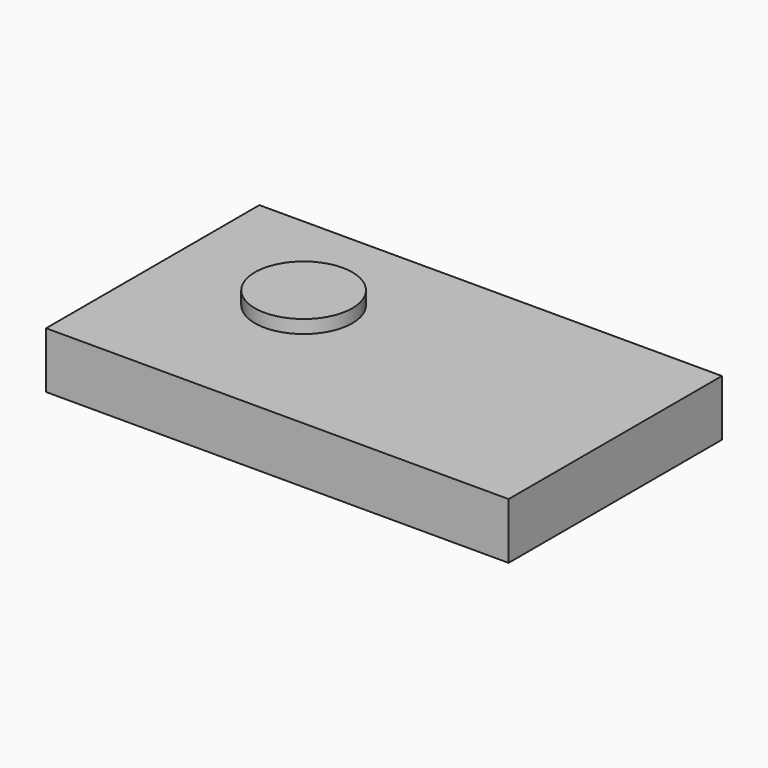
from build123d import *

# Parameters (mm, degrees)
F0_W     = 70
F0_H     = 40.35
F1_DEPTH = 8.5
F2_T     = -2
F3_R     = 7.375
F4_DEPTH = 2
F3_R_2   = 2.3617937204
F3_R_3   = 2.35
F5_DEPTH = 6


with BuildPart() as f1:
    # F0 (on Top) → F1 (new body)
    with BuildSketch(Plane.XY):
        with Locations((0, 20.175)):
            Rectangle(F0_W, F0_H)
    extrude(amount=F1_DEPTH)

    # F2
    f2_openings = [f1.faces().sort_by_distance(p)[0] for p in [
        (0, 20.175, 0),
    ]]
    offset(amount=F2_T, openings=f2_openings)


with BuildPart() as f4:
    # F3 (on face) → F4 (new body)
    with BuildSketch(Plane(origin=(0, 0, 6.5), x_dir=(1, 0, 0), z_dir=(0, 0, -1))):
        with Locations((-14.9081461403, -23.6036587987)):
            Circle(F3_R)
    extrude(amount=F4_DEPTH)

    # F5 (add): a face of the model
    f5_faces = [f4.faces().sort_by_distance(p)[0] for p in [
        (-14.9081461403, 23.6036587987, 4.5),
    ]]
    extrude(f5_faces, amount=-F5_DEPTH)


with BuildPart() as f4b:
    # F3 (on face) → F4, piece 2 (new body)
    with BuildSketch(Plane(origin=(0, 0, 6.5), x_dir=(1, 0, 0), z_dir=(0, 0, -1))):
        with BuildLine():
            ThreePointArc((7.6223985069, -23.715632426), (15.7731046859, -35.5022585988), (26.4967896861, -25.9964105162))
            ThreePointArc((26.4967896861, -25.9964105162), (26.2218277724, -23.7182716719), (25.4127340008, -21.5709738546))
            ThreePointArc((25.4127340008, -21.5709738546), (21.4016687656, -20.2961312745), (19.2148790784, -16.7000474618))
            ThreePointArc((19.2148790784, -16.7000474618), (16.8080721143, -16.4220858238), (14.4085460796, -16.7571339441))
            ThreePointArc((14.4085460796, -16.7571339441), (11.9640626624, -21.1614784837), (7.6223985069, -23.715632426))
        make_face()
        with Locations((16.9217896861, -25.9964105162)):
            Circle(F3_R_2, mode=Mode.SUBTRACT)
    extrude(amount=F4_DEPTH)


with BuildPart() as f4c:
    # F3 (on face) → F4, piece 3 (new body)
    with BuildSketch(Plane(origin=(0, 0, 6.5), x_dir=(1, 0, 0), z_dir=(0, 0, -1))):
        with BuildLine():
            ThreePointArc((19.2148790784, -16.7000474618), (22.8383196429, -18.4681106901), (25.4127340008, -21.5709738546))
            ThreePointArc((25.4127340008, -21.5709738546), (29.4578026559, -19.7125749443), (31.1091549004, -15.5786587987))
            ThreePointArc((31.1091549004, -15.5786587987), (24.5459741711, -9.6051483177), (19.2148790784, -16.7000474618))
        make_face()
    extrude(amount=F4_DEPTH)


with BuildPart() as f4d:
    # F3 (on face) → F4, piece 4 (new body)
    with BuildSketch(Plane(origin=(0, 0, 6.5), x_dir=(1, 0, 0), z_dir=(0, 0, -1))):
        with BuildLine():
            ThreePointArc((14.6841549004, -14.4763558539), (-2.4982405978, -8.6618774823), (7.6223985069, -23.715632426))
            ThreePointArc((7.6223985069, -23.715632426), (10.0668819241, -19.3112878864), (14.4085460796, -16.7571339441))
            ThreePointArc((14.4085460796, -16.7571339441), (14.6150029831, -15.6250408542), (14.6841549004, -14.4763558539))
        make_face()
        with Locations((5.1091549004, -14.4763558539)):
            Circle(F3_R_3, mode=Mode.SUBTRACT)
    extrude(amount=F4_DEPTH)


solid = Compound([f1.part, f4.part, f4b.part, f4c.part, f4d.part])
